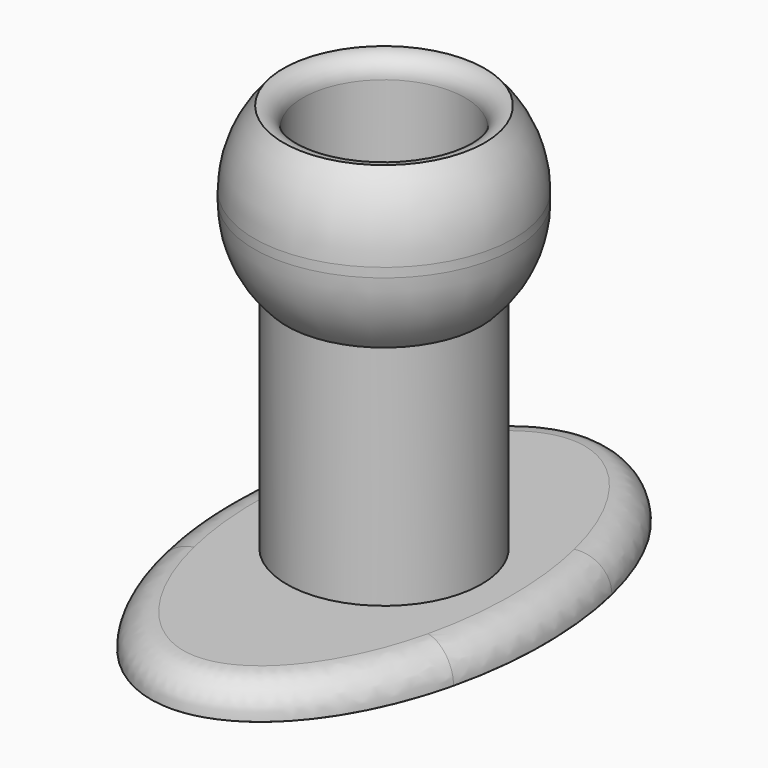
from build123d import *

# Parameters (mm, degrees)
F0_R     = 20
F0_R_2   = 15
F1_DEPTH = 5
F2_R     = 4.99999
F3_START = 40
F3_DEPTH = 25
F0_R_3   = 12.5
F4_DEPTH = 65
F5_R     = 3


# Not quite as in the source:
# - a fillet or chamfer that OpenCascade refuses, or shapes differently, is made with other operations: its cross-section is extruded or revolved along the edge and cut away or added
# - a fillet or chamfer is up to 0.001 mm smaller than in the source, because OpenCascade refuses the exact size


with BuildPart() as f1:
    # F0 (on Top) → F1 (new body)
    with BuildSketch(Plane.XY):
        with BuildLine():
            add(Edge.make_bspline(
                [(-22.8928557761, -15.2370323363), (-16.7035213729, -41.1210767925), (0, -41.1210767925)],
                knots=[5.091980066, 5.091980066, 5.091980066, 6.2831853072, 6.2831853072, 6.2831853072], degree=2, weights=[1, 0.8278105744, 1]))
            add(Edge.make_bspline(
                [(0, -41.1210767925), (16.7035213729, -41.1210767925), (22.8928557761, -15.2370323363)],
                knots=[0, 0, 0, 1.1912052412, 1.1912052412, 1.1912052412], degree=2, weights=[1, 0.8278105744, 1]))
            ThreePointArc((22.8928557761, -15.2370323363), (0, -27.5), (-22.8928557761, -15.2370323363))
        make_face()
        with BuildLine():
            ThreePointArc((-22.8928557761, 15.2370323363), (0, 27.5), (22.8928557761, 15.2370323363))
            add(Edge.make_bspline(
                [(22.8928557761, 15.2370323363), (0, 110.9758724176), (-22.8928557761, 15.2370323363)],
                knots=[1.9503874124, 1.9503874124, 1.9503874124, 4.3327978948, 4.3327978948, 4.3327978948], degree=2, weights=[1, 0.3705406941, 1]))
        make_face()
        with BuildLine():
            ThreePointArc((-22.8928557761, -15.2370323363), (0, -27.5), (22.8928557761, -15.2370323363))
            add(Edge.make_bspline(
                [(22.8928557761, -15.2370323363), (26.5363006249, 0), (22.8928557761, 15.2370323363)],
                knots=[1.1912052412, 1.1912052412, 1.1912052412, 1.9503874124, 1.9503874124, 1.9503874124], degree=2, weights=[1, 0.9288162326, 1]))
            ThreePointArc((22.8928557761, 15.2370323363), (0, 27.5), (-22.8928557761, 15.2370323363))
            add(Edge.make_bspline(
                [(-22.8928557761, 15.2370323363), (-26.5363006249, 0), (-22.8928557761, -15.2370323363)],
                knots=[4.3327978948, 4.3327978948, 4.3327978948, 5.091980066, 5.091980066, 5.091980066], degree=2, weights=[1, 0.9288162326, 1]))
        make_face()
        Circle(F0_R, mode=Mode.SUBTRACT)
        Circle(F0_R)
        Circle(F0_R_2, mode=Mode.SUBTRACT)
    extrude(amount=F1_DEPTH)

    # F2 (radius 5 in the source; OpenCascade refuses exactly that, so slightly less here)
    f2_edges = [f1.edges().sort_by_distance(p)[0] for p in [
        (-22.892856, 15.237032, 5),
    ]]
    fillet(f2_edges, radius=F2_R)



with BuildPart() as f3:
    # F0 (on Top) → F3 (new body)
    with BuildSketch(Plane.XY.offset(F3_START)):
        Circle(F0_R)
        Circle(F0_R_2, mode=Mode.SUBTRACT)
    extrude(amount=F3_DEPTH)


with BuildPart() as f1_1:
    add(f1.part)

    add(f3.part)  # F4 merges F3
    # F0 (on Top) → F4 (join)
    with BuildSketch(Plane.XY):
        Circle(F0_R_2)
        Circle(F0_R_3, mode=Mode.SUBTRACT)
    extrude(amount=F4_DEPTH)

    # F5
    f5_edges = [f1_1.edges().sort_by_distance(p)[0] for p in [
        (-12.5, 0, 65),
    ]]
    fillet(f5_edges, radius=F5_R)

    # F6: fillet of radius 17 on 3 edges, made by hand

    # F6_s1 → F6_t2 (revolve, cut)
    with BuildSketch(Plane.XZ):
        with BuildLine():
            ThreePointArc((20, 52.0415945788), (18.7003184681, 45.5223921736), (15, 40))
            Line((15, 40), (15.24, 39.7591681084))
            ThreePointArc((15.24, 39.7591681084), (17.5, 39.66), (20, 39.66))
            Line((20, 39.66), (20.34, 40))
            Line((20.34, 40), (20.34, 52.0415945788))
            Line((20.34, 52.0415945788), (20, 52.0415945788))
        make_face()
    revolve(axis=Axis((0, 0, 40), (0, 0, 1)), mode=Mode.SUBTRACT)

    # F6_s3 → F6_t4 (revolve, cut)
    with BuildSketch(Plane.XZ):
        with BuildLine():
            ThreePointArc((15.5, 65), (18.8350876221, 59.6629398166), (20, 53.4782813782))
            Line((20, 53.4782813782), (20.34, 53.4782813782))
            Line((20.34, 53.4782813782), (20.34, 65))
            Line((20.34, 65), (20, 65.34))
            ThreePointArc((20, 65.34), (17.75, 65.34), (15.75, 65.2304343724))
            Line((15.75, 65.2304343724), (15.5, 65))
        make_face()
    revolve(axis=Axis((0, 0, 65), (0, 0, 1)), mode=Mode.SUBTRACT)


solid = f1_1.part
